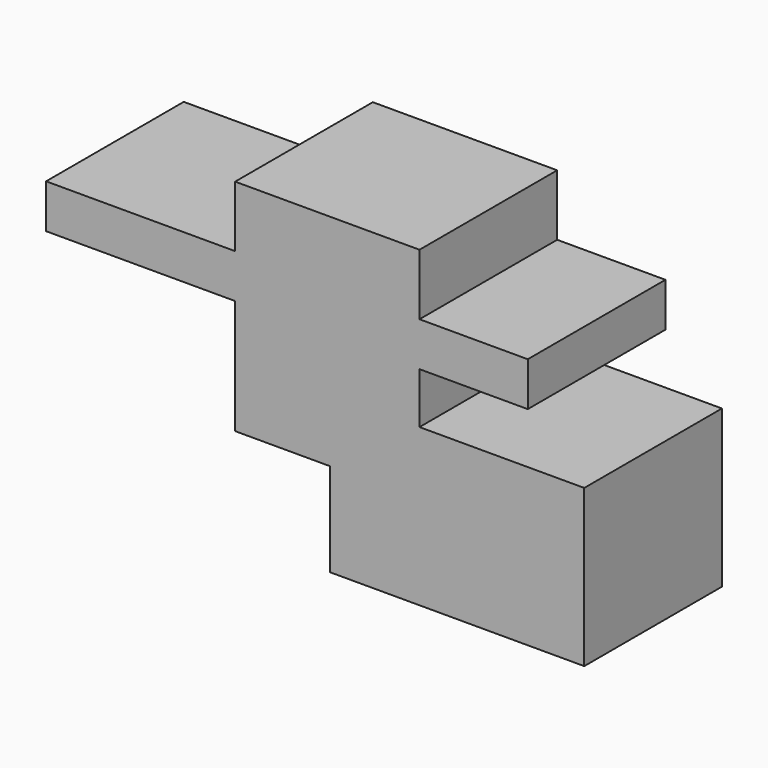
from build123d import *

# Parameters (mm, degrees)
F0_W     = 26.4005409554
F0_H     = 18.7582788058
F0_W_2   = 54.4221671298
F0_H_2   = 12.9686864093
F0_W_3   = 31.9585492834
F0_W_4   = 55.8116771281
F0_H_3   = 18.0635303259
F1_DEPTH = 25.4


with BuildPart() as f1:
    # F0 (on Front) → F1 (new body, symmetric)
    with BuildSketch(Plane.XZ):
        Polygon((-16.0769931972, -49.6410056949), (58.9561276138, -49.6410056949), (58.9561276138, -3.3242679201), (10.3235477582, -3.3242679201), (10.3235477582, -22.0825467259), (-16.0769931972, -22.0825467259), align=None)
        Polygon((-44.0986193717, -22.0825467259), (-16.0769931972, -22.0825467259), (-16.0769931972, -3.3242679201), (10.3235477582, -3.3242679201), (10.3235477582, 11.728673242), (-44.0986193717, 11.728673242), align=None)
        with Locations((-2.8767227195, -12.703407323)):
            Rectangle(F0_W, F0_H)
        with Locations((-16.8875358067, 18.2130164467)):
            Rectangle(F0_W_2, F0_H_2)
        with Locations((26.3028223999, 18.2130164467)):
            Rectangle(F0_W_3, F0_H_2)
        with Locations((-72.0044579357, 18.2130164467)):
            Rectangle(F0_W_4, F0_H_2)
        with Locations((-16.8875358067, 33.7291248143)):
            Rectangle(F0_W_2, F0_H_3)
    extrude(amount=F1_DEPTH, both=True)


solid = f1.part
